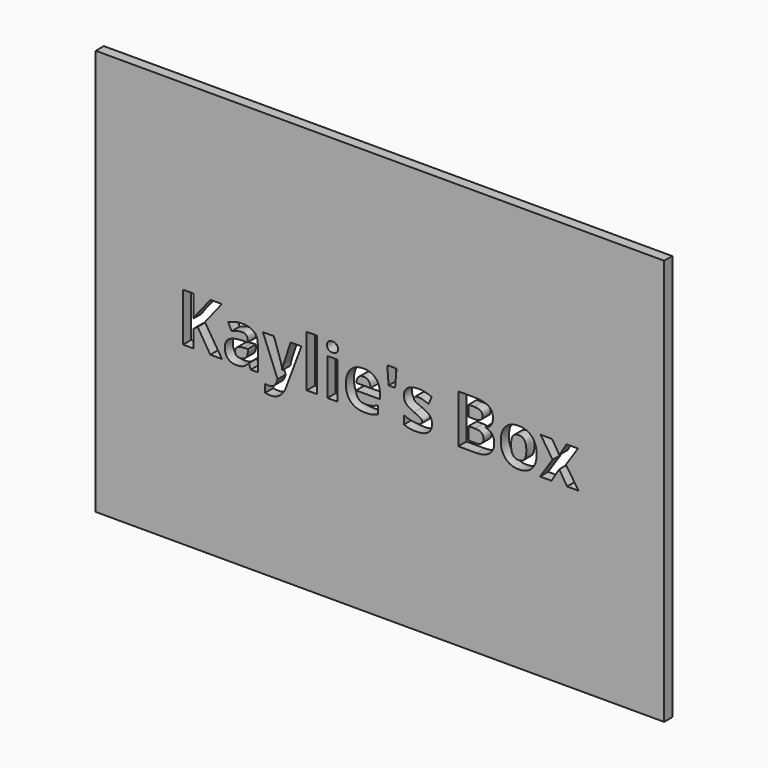
from build123d import *

# Parameters (mm, degrees)
F0_W         = 177.8
F0_H         = 127
F1_DEPTH     = 3.175
F2_TEXT_SIZE = 21.2008972821
F3_DEPTH     = 25.4


# Not quite as in the source:
# - Text() gives the source's letters only with a copy of the font that has no kerning and outlines rounded to 1/6400 em; it was checked with that copy


with BuildPart() as f1:
    # F0 (on Front) → F1 (new body)
    with BuildSketch(Plane.XZ):
        with Locations((-58.9783658773, 39.8776622713)):
            Rectangle(F0_W, F0_H)
    extrude(amount=F1_DEPTH)

    # F2 (on face) → F3 (cut)
    with BuildSketch(Plane.XZ.offset(3.175)):
        with Locations((-122.4783658773, 31.3320869393)):
            Text("Kaylie's Box", F2_TEXT_SIZE, font='Open Sans', font_style=FontStyle.BOLD, text_align=(TextAlign.LEFT, TextAlign.BOTTOM))
    extrude(amount=-F3_DEPTH, mode=Mode.SUBTRACT)


solid = f1.part
